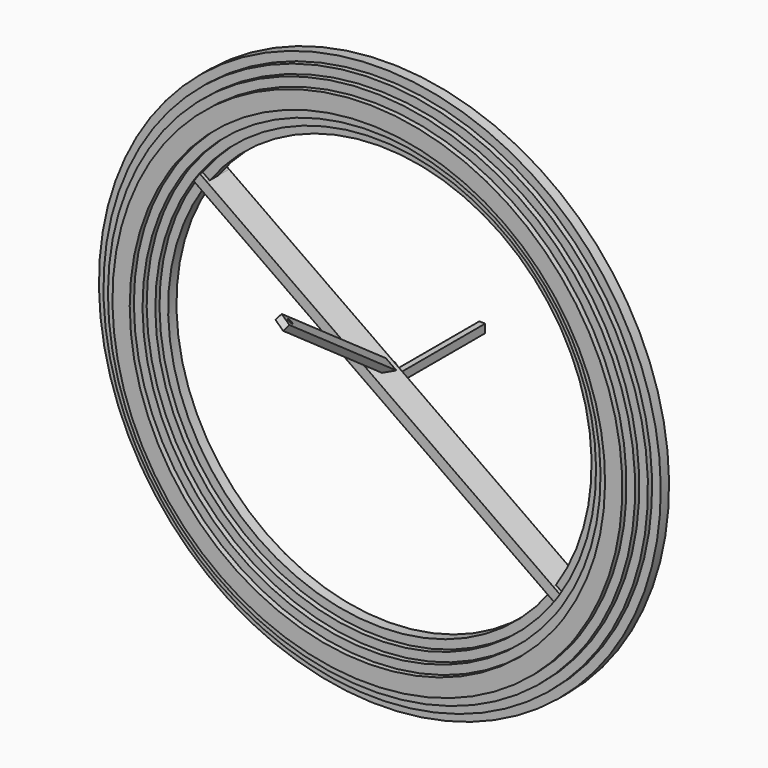
from build123d import *

# Parameters (mm, degrees)
F5_DEPTH  = 3
F6_DEPTH  = 4.5
F7_DEPTH  = 6
F8_DEPTH  = 7.5
F9_DEPTH  = 4
F12_W     = 1.7257919054
F12_H     = 2.4539034821
F13_DEPTH = 30
F15_W     = 3.5
F15_H     = 50
F16_DEPTH = 2
F17_R     = 0.7344979233
F18_DEPTH = 2


# Not quite as in the source:
# - the program builds the solid bodies; features that only make, move or delete a surface that nothing else refers to are left out


with BuildPart() as f5:
    # F4 (on 3pt) → F5 (new body)
    with BuildSketch(Plane.XZ):
        with BuildLine():
            ThreePointArc((-73.3595898483, 87.6719137514), (-53.6516810637, -25.4605484692), (59.4807811569, -5.7526396846))
            ThreePointArc((59.4807811569, -5.7526396846), (39.7728723723, 107.379822536), (-73.3595898483, 87.6719137514))
        make_face()
        with BuildLine():
            ThreePointArc((-71.3146702799, 86.2337538303), (38.3347124511, 105.3349029676), (57.4358615885, -4.3144797634))
            ThreePointArc((57.4358615885, -4.3144797634), (-52.2135211426, -23.4156289008), (-71.3146702799, 86.2337538303))
        make_face(mode=Mode.SUBTRACT)
    extrude(amount=F5_DEPTH)

    # F4 (on 3pt) → F6 (join)
    with BuildSketch(Plane.XZ):
        with BuildLine():
            ThreePointArc((-71.3146702799, 86.2337538303), (-52.2135211426, -23.4156289008), (57.4358615885, -4.3144797634))
            ThreePointArc((57.4358615885, -4.3144797634), (38.3347124511, 105.3349029676), (-71.3146702799, 86.2337538303))
        make_face()
        with BuildLine():
            ThreePointArc((-69.2697507115, 84.7955939091), (36.89655253, 103.2899833992), (55.3909420201, -2.8763198423))
            ThreePointArc((55.3909420201, -2.8763198423), (-50.7753612214, -21.3707093324), (-69.2697507115, 84.7955939091))
        make_face(mode=Mode.SUBTRACT)
    extrude(amount=F6_DEPTH)

    # F4 (on 3pt) → F7 (join)
    with BuildSketch(Plane.XZ):
        with BuildLine():
            ThreePointArc((-69.2697507115, 84.7955939091), (-50.7753612214, -21.3707093324), (55.3909420201, -2.8763198423))
            ThreePointArc((55.3909420201, -2.8763198423), (36.89655253, 103.2899833992), (-69.2697507115, 84.7955939091))
        make_face()
        with BuildLine():
            ThreePointArc((53.3460224517, -1.4381599211), (52.0519313936, -3.2209942256), (50.7051341625, -4.9643550723))
            ThreePointArc((50.7051341625, -4.9643550723), (-51.1200356047, -18.0316987059), (-67.2248311431, 83.357433988))
            ThreePointArc((-67.2248311431, 83.357433988), (35.4583926089, 101.2450638308), (53.3460224517, -1.4381599211))
        make_face(mode=Mode.SUBTRACT)
    extrude(amount=F7_DEPTH)



with BuildPart() as f5b:
    # F4 (on 3pt) → F5, piece 2 (new body)
    with BuildSketch(Plane.XZ):
        with BuildLine():
            ThreePointArc((46.0147924033, 5.5515923651), (29.7057529243, 93.0653855572), (-58.1678091893, 78.8215851838))
            Line((-58.1678091893, 78.8215851838), (-56.1222992763, 77.3830100825))
            ThreePointArc((-56.1222992763, 77.3830100825), (28.2675930031, 91.0204659888), (43.9692824902, 6.9901674664))
            Line((43.9692824902, 6.9901674664), (46.0147924033, 5.5515923651))
        make_face()
        with BuildLine():
            Line((-57.8480911816, 74.9291066004), (-59.8936010947, 76.3676817018))
            ThreePointArc((-59.8936010947, 76.3676817018), (-43.5845616157, -11.1461114904), (44.2890004979, 3.097688883))
            Line((44.2890004979, 3.097688883), (42.2434905848, 4.5362639843))
            ThreePointArc((42.2434905848, 4.5362639843), (-42.1464016945, -9.101191922), (-57.8480911816, 74.9291066004))
        make_face()
        with BuildLine():
            Line((-57.0002333011, 76.1666343822), (-59.0451528695, 77.6047943034))
            ThreePointArc((-59.0451528695, 77.6047943034), (-59.4730186996, 76.9887355996), (-59.8936010947, 76.3676817018))
            Line((-59.8936010947, 76.3676817018), (-57.8480911816, 74.9291066004))
            ThreePointArc((-57.8480911816, 74.9291066004), (-57.4279540232, 75.5504683256), (-57.0002333011, 76.1666343822))
        make_face()
        with BuildLine():
            ThreePointArc((-58.1678091893, 78.8215851838), (-58.6100629253, 78.2157724008), (-59.0451528695, 77.6047943034))
            Line((-59.0451528695, 77.6047943034), (-57.0002333011, 76.1666343822))
            ThreePointArc((-57.0002333011, 76.1666343822), (-56.5649932606, 76.7775122199), (-56.1222992763, 77.3830100825))
            Line((-56.1222992763, 77.3830100825), (-58.1678091893, 78.8215851838))
        make_face()
        with BuildLine():
            Line((42.2434905848, 4.5362639843), (44.2890004979, 3.097688883))
            ThreePointArc((44.2890004979, 3.097688883), (44.7312542339, 3.703501666), (45.1663441781, 4.3144797634))
            Line((45.1663441781, 4.3144797634), (43.1214246097, 5.7526396846))
            ThreePointArc((43.1214246097, 5.7526396846), (42.6861845692, 5.1417618469), (42.2434905848, 4.5362639843))
        make_face()
        with BuildLine():
            ThreePointArc((45.1663441781, 4.3144797634), (45.5942100081, 4.9305384673), (46.0147924033, 5.5515923651))
            Line((46.0147924033, 5.5515923651), (43.9692824902, 6.9901674664))
            ThreePointArc((43.9692824902, 6.9901674664), (43.5491453318, 6.3688057412), (43.1214246097, 5.7526396846))
            Line((43.1214246097, 5.7526396846), (45.1663441781, 4.3144797634))
        make_face()
    extrude(amount=F5_DEPTH)

    # F4 (on 3pt) → F6, piece 2 (join)
    with BuildSketch(Plane.XZ):
        with BuildLine():
            ThreePointArc((48.0602577115, 4.1130486336), (31.1439128454, 95.1103051256), (-60.2132744976, 80.2601289153))
            Line((-60.2132744976, 80.2601289153), (-58.1678091893, 78.8215851838))
            ThreePointArc((-58.1678091893, 78.8215851838), (29.7057529243, 93.0653855572), (46.0147924033, 5.5515923651))
            Line((46.0147924033, 5.5515923651), (48.0602577115, 4.1130486336))
        make_face()
        with BuildLine():
            Line((-59.0451528695, 77.6047943034), (-61.0900724379, 79.0429542245))
            ThreePointArc((-61.0900724379, 79.0429542245), (-61.5180724997, 78.4269946351), (-61.9390664029, 77.8062254332))
            Line((-61.9390664029, 77.8062254332), (-59.8936010947, 76.3676817018))
            ThreePointArc((-59.8936010947, 76.3676817018), (-59.4730186996, 76.9887355996), (-59.0451528695, 77.6047943034))
        make_face()
        with BuildLine():
            ThreePointArc((-60.2132744976, 80.2601289153), (-60.6551211593, 79.6540251319), (-61.0900724379, 79.0429542245))
            Line((-61.0900724379, 79.0429542245), (-59.0451528695, 77.6047943034))
            ThreePointArc((-59.0451528695, 77.6047943034), (-58.6100629253, 78.2157724008), (-58.1678091893, 78.8215851838))
            Line((-58.1678091893, 78.8215851838), (-60.2132744976, 80.2601289153))
        make_face()
        with BuildLine():
            Line((-59.8936010947, 76.3676817018), (-61.9390664029, 77.8062254332))
            ThreePointArc((-61.9390664029, 77.8062254332), (-45.0227215368, -13.1910310588), (46.3344658061, 1.6591451516))
            Line((46.3344658061, 1.6591451516), (44.2890004979, 3.097688883))
            ThreePointArc((44.2890004979, 3.097688883), (-43.5845616157, -11.1461114904), (-59.8936010947, 76.3676817018))
        make_face()
        with BuildLine():
            Line((44.2890004979, 3.097688883), (46.3344658061, 1.6591451516))
            ThreePointArc((46.3344658061, 1.6591451516), (46.7763124678, 2.2652489349), (47.2112637465, 2.8763198423))
            Line((47.2112637465, 2.8763198423), (45.1663441781, 4.3144797634))
            ThreePointArc((45.1663441781, 4.3144797634), (44.7312542339, 3.703501666), (44.2890004979, 3.097688883))
        make_face()
        with BuildLine():
            ThreePointArc((47.2112637465, 2.8763198423), (47.6392638082, 3.4922794317), (48.0602577115, 4.1130486336))
            Line((48.0602577115, 4.1130486336), (46.0147924033, 5.5515923651))
            ThreePointArc((46.0147924033, 5.5515923651), (45.5942100081, 4.9305384673), (45.1663441781, 4.3144797634))
            Line((45.1663441781, 4.3144797634), (47.2112637465, 2.8763198423))
        make_face()
    extrude(amount=F6_DEPTH)

    # F4 (on 3pt) → F7, piece 2 (join)
    with BuildSketch(Plane.XZ):
        with BuildLine():
            ThreePointArc((50.1056832868, 2.6745328458), (32.5820727666, 97.155224694), (-62.2587000728, 81.6986447031))
            Line((-62.2587000728, 81.6986447031), (-60.2132744976, 80.2601289153))
            ThreePointArc((-60.2132744976, 80.2601289153), (31.1439128454, 95.1103051256), (48.0602577115, 4.1130486336))
            Line((48.0602577115, 4.1130486336), (50.1056832868, 2.6745328458))
        make_face()
        with BuildLine():
            Line((46.5367490505, 1.5168825123), (48.3798913814, 0.2206293637))
            ThreePointArc((48.3798913814, 0.2206293637), (48.821360529, 0.8270028531), (49.2561833149, 1.4381599211))
            Line((49.2561833149, 1.4381599211), (47.2112637465, 2.8763198423))
            ThreePointArc((47.2112637465, 2.8763198423), (46.8221297031, 2.2223409394), (46.5367490505, 1.5168825123))
        make_face()
        with BuildLine():
            ThreePointArc((49.2561833149, 1.4381599211), (49.6843079108, 2.0540277213), (50.1056832868, 2.6745328458))
            Line((50.1056832868, 2.6745328458), (48.0602577115, 4.1130486336))
            ThreePointArc((48.0602577115, 4.1130486336), (47.6392638082, 3.4922794317), (47.2112637465, 2.8763198423))
            Line((47.2112637465, 2.8763198423), (49.2561833149, 1.4381599211))
        make_face()
        with BuildLine():
            Line((-61.9390664029, 77.8062254332), (-63.9844919782, 79.244741221))
            ThreePointArc((-63.9844919782, 79.244741221), (-47.5792051598, -14.432580971), (46.7028109016, -1.9635964074))
            ThreePointArc((46.7028109016, -1.9635964074), (46.3067843573, -0.2382907061), (46.5367490505, 1.5168825123))
            Line((46.5367490505, 1.5168825123), (46.3344658061, 1.6591451516))
            ThreePointArc((46.3344658061, 1.6591451516), (-45.0227215368, -13.1910310588), (-61.9390664029, 77.8062254332))
        make_face()
        with BuildLine():
            ThreePointArc((46.5367490505, 1.5168825123), (46.3067843573, -0.2382907061), (46.7028109016, -1.9635964074))
            ThreePointArc((46.7028109016, -1.9635964074), (47.552296206, -0.8798873024), (48.3798913814, 0.2206293637))
            Line((48.3798913814, 0.2206293637), (46.5367490505, 1.5168825123))
        make_face()
        with BuildLine():
            Line((46.3344658061, 1.6591451516), (46.5367490505, 1.5168825123))
            ThreePointArc((46.5367490505, 1.5168825123), (46.8221297031, 2.2223409394), (47.2112637465, 2.8763198423))
            ThreePointArc((47.2112637465, 2.8763198423), (46.7763124678, 2.2652489349), (46.3344658061, 1.6591451516))
        make_face()
        with BuildLine():
            ThreePointArc((-62.2587000728, 81.6986447031), (-62.7001692204, 81.0922712137), (-63.1349920063, 80.4811141457))
            Line((-63.1349920063, 80.4811141457), (-61.0900724379, 79.0429542245))
            ThreePointArc((-61.0900724379, 79.0429542245), (-60.6551211593, 79.6540251319), (-60.2132744976, 80.2601289153))
            Line((-60.2132744976, 80.2601289153), (-62.2587000728, 81.6986447031))
        make_face()
        with BuildLine():
            Line((-61.0900724379, 79.0429542245), (-63.1349920063, 80.4811141457))
            ThreePointArc((-63.1349920063, 80.4811141457), (-63.5631166022, 79.8652463455), (-63.9844919782, 79.244741221))
            Line((-63.9844919782, 79.244741221), (-61.9390664029, 77.8062254332))
            ThreePointArc((-61.9390664029, 77.8062254332), (-61.5180724997, 78.4269946351), (-61.0900724379, 79.0429542245))
        make_face()
    extrude(amount=F7_DEPTH)


with BuildPart() as f5_1:
    add(f5.part)

    add(f5b.part)  # F8 merges F5b
    # F4 (on 3pt) → F8 (join)
    with BuildSketch(Plane.XZ):
        with BuildLine():
            ThreePointArc((-67.2248311431, 83.357433988), (-51.1200356047, -18.0316987059), (50.7051341625, -4.9643550723))
            ThreePointArc((50.7051341625, -4.9643550723), (52.0519313936, -3.2209942256), (53.3460224517, -1.4381599211))
            ThreePointArc((53.3460224517, -1.4381599211), (35.4583926089, 101.2450638308), (-67.2248311431, 83.357433988))
        make_face()
        with BuildLine():
            add(Edge.make_bspline(
                [(-67.6660389606, 81.6562709846), (-67.6145472876, 81.1695281785), (-66.3966172272, 81.0419899879)],
                knots=[0, 0, 0, 1.0228935043, 1.0228935043, 1.0228935043], degree=2, weights=[1, 0.8720373231, 1]))
            add(Edge.make_bspline(
                [(-66.5532444111, 82.5225624891), (-67.7175306335, 82.1430137906), (-67.6660389606, 81.6562709846)],
                knots=[5.2602918029, 5.2602918029, 5.2602918029, 6.2831853072, 6.2831853072, 6.2831853072], degree=2, weights=[1, 0.8720373231, 1]))
            ThreePointArc((-66.5532444111, 82.5225624891), (-65.582869931, 83.3641355007), (-64.317015622, 83.1462258079))
            Line((-64.317015622, 83.1462258079), (-64.3040901023, 83.1371354922))
            ThreePointArc((-64.3040901023, 83.1371354922), (34.0202326877, 99.2001442624), (52.1510733163, 1.2360420567))
            Line((52.1510733163, 1.2360420567), (52.163998836, 1.226951741))
            ThreePointArc((52.163998836, 1.226951741), (52.5280546243, -0.8628959527), (50.4382069306, -1.226951741))
            Line((50.4382069306, -1.226951741), (50.4252814109, -1.2178614254))
            ThreePointArc((50.4252814109, -1.2178614254), (49.3711347658, -2.6152609375), (48.2829556417, -3.9863250279))
            ThreePointArc((48.2829556417, -3.9863250279), (-49.3183384503, -16.2563964918), (-66.0298820077, 80.6832320101))
            Line((-66.0298820077, 80.6832320101), (-66.0428075274, 80.6923223258))
            ThreePointArc((-66.0428075274, 80.6923223258), (-66.2343083584, 80.8523872769), (-66.3966172272, 81.0419899879))
        make_face(mode=Mode.SUBTRACT)
        with BuildLine():
            Line((-64.3040901023, 83.1371354922), (-63.7890663874, 82.7749273757))
            add(Edge.make_bspline(
                [(-62.7179712727, 82.0216429486), (-62.4931072818, 82.5873668381), (-63.7890663874, 82.7749273757)],
                knots=[2.9603434797, 2.9603434797, 2.9603434797, 4.0822497642, 4.0822497642, 4.0822497642], degree=2, weights=[1, 0.8467484302, 1]))
            Line((-62.7179712727, 82.0216429486), (-62.2587000728, 81.6986447031))
            ThreePointArc((-62.2587000728, 81.6986447031), (32.5820727666, 97.155224694), (50.1056832868, 2.6745328458))
            Line((50.1056832868, 2.6745328458), (52.1510733163, 1.2360420567))
            ThreePointArc((52.1510733163, 1.2360420567), (34.0202326877, 99.2001442624), (-64.3040901023, 83.1371354922))
        make_face()
        with BuildLine():
            Line((-63.9844919782, 79.244741221), (-66.0298820077, 80.6832320101))
            ThreePointArc((-66.0298820077, 80.6832320101), (-49.3183384503, -16.2563964918), (48.2829556417, -3.9863250279))
            ThreePointArc((48.2829556417, -3.9863250279), (47.3608751769, -3.0780847327), (46.7028109016, -1.9635964074))
            ThreePointArc((46.7028109016, -1.9635964074), (-47.5792051598, -14.432580971), (-63.9844919782, 79.244741221))
        make_face()
        with BuildLine():
            ThreePointArc((46.7028109016, -1.9635964074), (47.3608751769, -3.0780847327), (48.2829556417, -3.9863250279))
            ThreePointArc((48.2829556417, -3.9863250279), (49.3711347658, -2.6152609375), (50.4252814109, -1.2178614254))
            Line((50.4252814109, -1.2178614254), (48.3798913814, 0.2206293637))
            ThreePointArc((48.3798913814, 0.2206293637), (47.552296206, -0.8798873024), (46.7028109016, -1.9635964074))
        make_face()
        with BuildLine():
            Line((48.3798913814, 0.2206293637), (50.4252814109, -1.2178614254))
            ThreePointArc((50.4252814109, -1.2178614254), (50.8663994972, -0.6112372691), (51.3011028833, 0))
            Line((51.3011028833, 0), (49.2561833149, 1.4381599211))
            ThreePointArc((49.2561833149, 1.4381599211), (48.821360529, 0.8270028531), (48.3798913814, 0.2206293637))
        make_face()
        with BuildLine():
            ThreePointArc((51.3011028833, 0), (51.7293433302, 0.615782553), (52.1510733163, 1.2360420567))
            Line((52.1510733163, 1.2360420567), (50.1056832868, 2.6745328458))
            ThreePointArc((50.1056832868, 2.6745328458), (49.6843079108, 2.0540277213), (49.2561833149, 1.4381599211))
            Line((49.2561833149, 1.4381599211), (51.3011028833, 0))
        make_face()
        with BuildLine():
            Line((52.163998836, 1.226951741), (52.1510733163, 1.2360420567))
            ThreePointArc((52.1510733163, 1.2360420567), (51.7293433302, 0.615782553), (51.3011028833, 0))
            ThreePointArc((51.3011028833, 0), (50.8663994972, -0.6112372691), (50.4252814109, -1.2178614254))
            Line((50.4252814109, -1.2178614254), (50.4382069306, -1.226951741))
            ThreePointArc((50.4382069306, -1.226951741), (52.5280546243, -0.8628959527), (52.163998836, 1.226951741))
        make_face()
        with BuildLine():
            add(Edge.make_bspline(
                [(-65.8068258149, 81.0130418546), (-64.9669181483, 81.013935447), (-64.1732309553, 81.2112913458)],
                knots=[1.2791714406, 1.2791714406, 1.2791714406, 1.9505002951, 1.9505002951, 1.9505002951], degree=2, weights=[1, 0.944191658, 1]))
            ThreePointArc((-65.8068258149, 81.0130418546), (-65.9185844476, 80.8482928481), (-66.0298820077, 80.6832320101))
            Line((-66.0298820077, 80.6832320101), (-63.9844919782, 79.244741221))
            ThreePointArc((-63.9844919782, 79.244741221), (-63.5631166022, 79.8652463455), (-63.1349920063, 80.4811141457))
            Line((-63.1349920063, 80.4811141457), (-64.1732309553, 81.2112913458))
        make_face()
        with BuildLine():
            add(Edge.make_bspline(
                [(-63.7890663874, 82.7749273757), (-64.1322743412, 82.8245989032), (-64.5319262057, 82.8254939338)],
                knots=[4.0822497642, 4.0822497642, 4.0822497642, 4.4120018269, 4.4120018269, 4.4120018269], degree=2, weights=[1, 0.9864387099, 1]))
            ThreePointArc((-64.5319262057, 82.8254939338), (-64.8576913162, 82.3736513595), (-65.1799115747, 81.9192740668))
            Line((-65.1799115747, 81.9192740668), (-64.1732309553, 81.2112913458))
            add(Edge.make_bspline(
                [(-64.1732309553, 81.2112913458), (-62.915789112, 81.5239630979), (-62.7179712727, 82.0216429486)],
                knots=[1.9505002951, 1.9505002951, 1.9505002951, 2.9603434797, 2.9603434797, 2.9603434797], degree=2, weights=[1, 0.875212406, 1]))
            Line((-62.7179712727, 82.0216429486), (-63.7890663874, 82.7749273757))
        make_face()
        with BuildLine():
            ThreePointArc((-66.5532444111, 82.5225624891), (-66.6715880062, 81.7614722175), (-66.3966172272, 81.0419899879))
            add(Edge.make_bspline(
                [(-66.3966172272, 81.0419899879), (-66.1170245039, 81.0127118288), (-65.8068258149, 81.0130418546)],
                knots=[1.0228935043, 1.0228935043, 1.0228935043, 1.2791714406, 1.2791714406, 1.2791714406], degree=2, weights=[1, 0.9918014297, 1]))
            ThreePointArc((-65.8068258149, 81.0130418546), (-65.4951218735, 81.4673707765), (-65.1799115747, 81.9192740668))
            ThreePointArc((-65.1799115747, 81.9192740668), (-64.8576913162, 82.3736513595), (-64.5319262057, 82.8254939338))
            add(Edge.make_bspline(
                [(-64.5319262057, 82.8254939338), (-65.616534656, 82.8279229421), (-66.5532444111, 82.5225624891)],
                knots=[4.4120018269, 4.4120018269, 4.4120018269, 5.2602918029, 5.2602918029, 5.2602918029], degree=2, weights=[1, 0.9113909391, 1]))
        make_face()
        with BuildLine():
            add(Edge.make_bspline(
                [(-64.1732309553, 81.2112913458), (-62.915789112, 81.5239630979), (-62.7179712727, 82.0216429486)],
                knots=[1.9505002951, 1.9505002951, 1.9505002951, 2.9603434797, 2.9603434797, 2.9603434797], degree=2, weights=[1, 0.875212406, 1]))
            Line((-64.1732309553, 81.2112913458), (-63.1349920063, 80.4811141457))
            ThreePointArc((-63.1349920063, 80.4811141457), (-62.7001692204, 81.0922712137), (-62.2587000728, 81.6986447031))
            Line((-62.2587000728, 81.6986447031), (-62.7179712727, 82.0216429486))
        make_face()
        with BuildLine():
            ThreePointArc((-64.317015622, 83.1462258079), (-65.582869931, 83.3641355007), (-66.5532444111, 82.5225624891))
            add(Edge.make_bspline(
                [(-64.5319262057, 82.8254939338), (-65.616534656, 82.8279229421), (-66.5532444111, 82.5225624891)],
                knots=[4.4120018269, 4.4120018269, 4.4120018269, 5.2602918029, 5.2602918029, 5.2602918029], degree=2, weights=[1, 0.9113909391, 1]))
            ThreePointArc((-64.5319262057, 82.8254939338), (-64.4182193637, 82.981469125), (-64.3040901023, 83.1371354922))
            Line((-64.3040901023, 83.1371354922), (-64.317015622, 83.1462258079))
        make_face()
        with BuildLine():
            add(Edge.make_bspline(
                [(-66.5532444111, 82.5225624891), (-67.7175306335, 82.1430137906), (-67.6660389606, 81.6562709846)],
                knots=[5.2602918029, 5.2602918029, 5.2602918029, 6.2831853072, 6.2831853072, 6.2831853072], degree=2, weights=[1, 0.8720373231, 1]))
            add(Edge.make_bspline(
                [(-67.6660389606, 81.6562709846), (-67.6145472876, 81.1695281785), (-66.3966172272, 81.0419899879)],
                knots=[0, 0, 0, 1.0228935043, 1.0228935043, 1.0228935043], degree=2, weights=[1, 0.8720373231, 1]))
            ThreePointArc((-66.3966172272, 81.0419899879), (-66.6715880062, 81.7614722175), (-66.5532444111, 82.5225624891))
        make_face()
        with BuildLine():
            ThreePointArc((-65.1799115747, 81.9192740668), (-65.4951218735, 81.4673707765), (-65.8068258149, 81.0130418546))
            add(Edge.make_bspline(
                [(-65.8068258149, 81.0130418546), (-64.9669181483, 81.013935447), (-64.1732309553, 81.2112913458)],
                knots=[1.2791714406, 1.2791714406, 1.2791714406, 1.9505002951, 1.9505002951, 1.9505002951], degree=2, weights=[1, 0.944191658, 1]))
            Line((-64.1732309553, 81.2112913458), (-65.1799115747, 81.9192740668))
        make_face()
        with BuildLine():
            add(Edge.make_bspline(
                [(-62.7179712727, 82.0216429486), (-62.4931072818, 82.5873668381), (-63.7890663874, 82.7749273757)],
                knots=[2.9603434797, 2.9603434797, 2.9603434797, 4.0822497642, 4.0822497642, 4.0822497642], degree=2, weights=[1, 0.8467484302, 1]))
            Line((-63.7890663874, 82.7749273757), (-62.7179712727, 82.0216429486))
        make_face()
        with BuildLine():
            ThreePointArc((-64.3040901023, 83.1371354922), (-64.4182193637, 82.981469125), (-64.5319262057, 82.8254939338))
            add(Edge.make_bspline(
                [(-63.7890663874, 82.7749273757), (-64.1322743412, 82.8245989032), (-64.5319262057, 82.8254939338)],
                knots=[4.0822497642, 4.0822497642, 4.0822497642, 4.4120018269, 4.4120018269, 4.4120018269], degree=2, weights=[1, 0.9864387099, 1]))
            Line((-63.7890663874, 82.7749273757), (-64.3040901023, 83.1371354922))
        make_face()
        with BuildLine():
            add(Edge.make_bspline(
                [(-66.3966172272, 81.0419899879), (-66.1170245039, 81.0127118288), (-65.8068258149, 81.0130418546)],
                knots=[1.0228935043, 1.0228935043, 1.0228935043, 1.2791714406, 1.2791714406, 1.2791714406], degree=2, weights=[1, 0.9918014297, 1]))
            ThreePointArc((-66.3966172272, 81.0419899879), (-66.2343083584, 80.8523872769), (-66.0428075274, 80.6923223258))
            Line((-66.0428075274, 80.6923223258), (-66.0298820077, 80.6832320101))
            ThreePointArc((-66.0298820077, 80.6832320101), (-65.9185844476, 80.8482928481), (-65.8068258149, 81.0130418546))
        make_face()
    extrude(amount=F8_DEPTH)

    # F4 (on 3pt) → F9 (join, symmetric)
    with BuildSketch(Plane.XZ):
        with BuildLine():
            ThreePointArc((-56.1222992763, 77.3830100825), (-56.5649932606, 76.7775122199), (-57.0002333011, 76.1666343822))
            Line((-57.0002333011, 76.1666343822), (43.1214246097, 5.7526396846))
            ThreePointArc((43.1214246097, 5.7526396846), (43.5491453318, 6.3688057412), (43.9692824902, 6.9901674664))
            Line((43.9692824902, 6.9901674664), (-56.1222992763, 77.3830100825))
        make_face()
        with BuildLine():
            Line((43.1214246097, 5.7526396846), (-57.0002333011, 76.1666343822))
            ThreePointArc((-57.0002333011, 76.1666343822), (-57.4279540232, 75.5504683256), (-57.8480911816, 74.9291066004))
            Line((-57.8480911816, 74.9291066004), (42.2434905848, 4.5362639843))
            ThreePointArc((42.2434905848, 4.5362639843), (42.6861845692, 5.1417618469), (43.1214246097, 5.7526396846))
        make_face()
        with BuildLine():
            Line((44.2890004979, 3.097688883), (46.3344658061, 1.6591451516))
            ThreePointArc((46.3344658061, 1.6591451516), (46.7763124678, 2.2652489349), (47.2112637465, 2.8763198423))
            Line((47.2112637465, 2.8763198423), (45.1663441781, 4.3144797634))
            ThreePointArc((45.1663441781, 4.3144797634), (44.7312542339, 3.703501666), (44.2890004979, 3.097688883))
        make_face()
        with BuildLine():
            Line((42.2434905848, 4.5362639843), (44.2890004979, 3.097688883))
            ThreePointArc((44.2890004979, 3.097688883), (44.7312542339, 3.703501666), (45.1663441781, 4.3144797634))
            Line((45.1663441781, 4.3144797634), (43.1214246097, 5.7526396846))
            ThreePointArc((43.1214246097, 5.7526396846), (42.6861845692, 5.1417618469), (42.2434905848, 4.5362639843))
        make_face()
        with BuildLine():
            ThreePointArc((45.1663441781, 4.3144797634), (45.5942100081, 4.9305384673), (46.0147924033, 5.5515923651))
            Line((46.0147924033, 5.5515923651), (43.9692824902, 6.9901674664))
            ThreePointArc((43.9692824902, 6.9901674664), (43.5491453318, 6.3688057412), (43.1214246097, 5.7526396846))
            Line((43.1214246097, 5.7526396846), (45.1663441781, 4.3144797634))
        make_face()
        with BuildLine():
            ThreePointArc((47.2112637465, 2.8763198423), (47.6392638082, 3.4922794317), (48.0602577115, 4.1130486336))
            Line((48.0602577115, 4.1130486336), (46.0147924033, 5.5515923651))
            ThreePointArc((46.0147924033, 5.5515923651), (45.5942100081, 4.9305384673), (45.1663441781, 4.3144797634))
            Line((45.1663441781, 4.3144797634), (47.2112637465, 2.8763198423))
        make_face()
        with BuildLine():
            ThreePointArc((-58.1678091893, 78.8215851838), (-58.6100629253, 78.2157724008), (-59.0451528695, 77.6047943034))
            Line((-59.0451528695, 77.6047943034), (-57.0002333011, 76.1666343822))
            ThreePointArc((-57.0002333011, 76.1666343822), (-56.5649932606, 76.7775122199), (-56.1222992763, 77.3830100825))
            Line((-56.1222992763, 77.3830100825), (-58.1678091893, 78.8215851838))
        make_face()
        with BuildLine():
            Line((-57.0002333011, 76.1666343822), (-59.0451528695, 77.6047943034))
            ThreePointArc((-59.0451528695, 77.6047943034), (-59.4730186996, 76.9887355996), (-59.8936010947, 76.3676817018))
            Line((-59.8936010947, 76.3676817018), (-57.8480911816, 74.9291066004))
            ThreePointArc((-57.8480911816, 74.9291066004), (-57.4279540232, 75.5504683256), (-57.0002333011, 76.1666343822))
        make_face()
        with BuildLine():
            ThreePointArc((-60.2132744976, 80.2601289153), (-60.6551211593, 79.6540251319), (-61.0900724379, 79.0429542245))
            Line((-61.0900724379, 79.0429542245), (-59.0451528695, 77.6047943034))
            ThreePointArc((-59.0451528695, 77.6047943034), (-58.6100629253, 78.2157724008), (-58.1678091893, 78.8215851838))
            Line((-58.1678091893, 78.8215851838), (-60.2132744976, 80.2601289153))
        make_face()
        with BuildLine():
            Line((-59.0451528695, 77.6047943034), (-61.0900724379, 79.0429542245))
            ThreePointArc((-61.0900724379, 79.0429542245), (-61.5180724997, 78.4269946351), (-61.9390664029, 77.8062254332))
            Line((-61.9390664029, 77.8062254332), (-59.8936010947, 76.3676817018))
            ThreePointArc((-59.8936010947, 76.3676817018), (-59.4730186996, 76.9887355996), (-59.0451528695, 77.6047943034))
        make_face()
    extrude(amount=F9_DEPTH, both=True)

    # F12 (on face) → F13 (join)
    with BuildSketch(Plane(origin=(0, 4, 0), x_dir=(-1, 0, 0), z_dir=(0, 1, 0))):
        with Locations((6.9394043457, 40.9596370334)):
            Rectangle(F12_W, F12_H)
    extrude(amount=F13_DEPTH)

    # F15 (on face) → F16 (join)
    with BuildSketch(Plane(origin=(13.0819673587, 13.1294115227, 18.6012491737), x_dir=(0.8670660442, -0.2872867724, -0.4070169351), z_dir=(0.4981932106, 0.5, 0.708380918))):
        with Locations((-25.8361325358, -44.6442002186)):
            Rectangle(F15_W, F15_H)
    extrude(amount=F16_DEPTH)

    # F17 (on face) → F18 (cut, through all)
    with BuildSketch(Plane(origin=(13.0819673587, 13.1294115227, 18.6012491737), x_dir=(0.8670660442, -0.2872867724, -0.4070169351), z_dir=(-0.4981932106, -0.5, -0.708380918))):
        with Locations((-25.8361325358, 67.6442002186)):
            Circle(F17_R)
    extrude(amount=-F18_DEPTH, mode=Mode.SUBTRACT)


solid = f5_1.part
